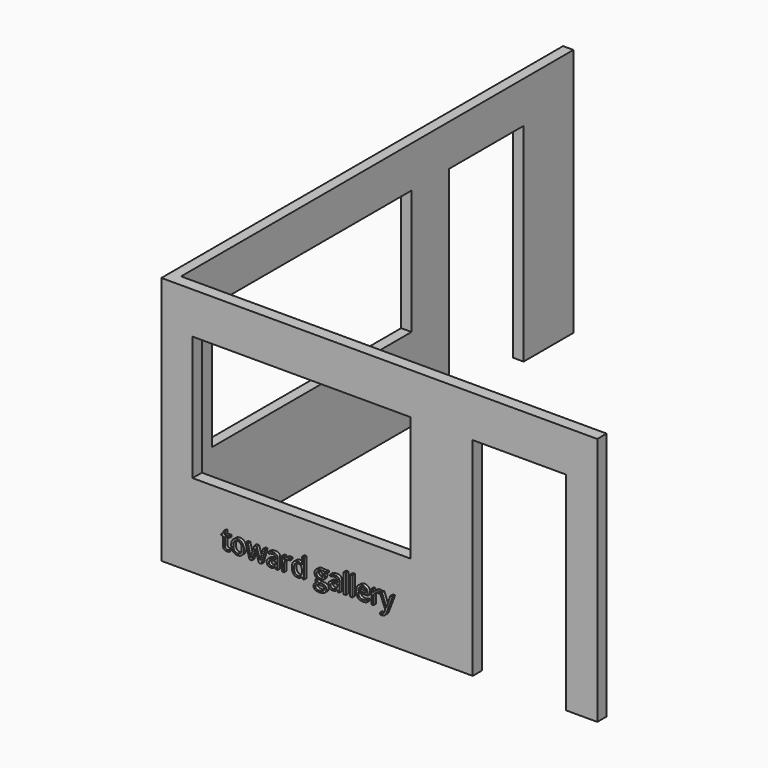
from build123d import *

# Parameters (mm, degrees)
F0_W          = 4267.2
F0_H          = 2438.4
F1_DEPTH      = 114.3
F2_W          = 914.4
F2_H          = 2032
F3_DEPTH      = 114.301
F4_W          = 2133.6
F4_H          = 1219.2
F5_DEPTH      = 114.301
F6_W          = 101.6
F6_H          = 2438.4
F7_DEPTH      = 4800.6
F8_W          = 914.4
F8_H          = 2032.1016
F8_W_2        = 2438.4
F8_H_2        = 1219.2
F9_DEPTH      = 101.601
F10_TEXT_SIZE = 253.0523886283
F11_DEPTH     = 30.48


# Not quite as in the source:
# - Text() gives the source's letters only with a copy of the font that has no kerning and outlines rounded to 1/6400 em; it was checked with that copy


with BuildPart() as f1:
    # F0 (on Front) → F1 (new body)
    with BuildSketch(Plane.XZ):
        with Locations((2133.6, 1219.2)):
            Rectangle(F0_W, F0_H)
    extrude(amount=F1_DEPTH)

    # F2 (on face) → F3 (cut, through all)
    with BuildSketch(Plane.XZ.offset(114.3)):
        with Locations((3505.2, 1016)):
            Rectangle(F2_W, F2_H)
    extrude(amount=-F3_DEPTH, mode=Mode.SUBTRACT)

    # F4 (on face) → F5 (cut, through all)
    with BuildSketch(Plane.XZ.offset(114.3)):
        with Locations((1371.6, 1422.4)):
            Rectangle(F4_W, F4_H)
    extrude(amount=-F5_DEPTH, mode=Mode.SUBTRACT)

    # F6 (on face) → F7 (join)
    with BuildSketch(Plane(origin=(0, 0, 0), x_dir=(-1, 0, 0), z_dir=(0, 1, 0))):
        with Locations((-50.8, 1219.2)):
            Rectangle(F6_W, F6_H)
    extrude(amount=F7_DEPTH)

    # F8 (on face) → F9 (cut, through all)
    with BuildSketch(Plane.YZ.offset(101.6)):
        with Locations((3733.8, 1016.0508)):
            Rectangle(F8_W, F8_H)
        with Locations((1600.2, 1422.5016)):
            Rectangle(F8_W_2, F8_H_2)
    extrude(amount=-F9_DEPTH, mode=Mode.SUBTRACT)

    # F10 (on face) → F11 (join)
    with BuildSketch(Plane.XZ.offset(114.3)):
        with Locations((604.3486595154, 312.6853406429)):
            Text('toward gallery', F10_TEXT_SIZE, font='Open Sans', text_align=(TextAlign.LEFT, TextAlign.BOTTOM))
    extrude(amount=F11_DEPTH)


solid = f1.part
